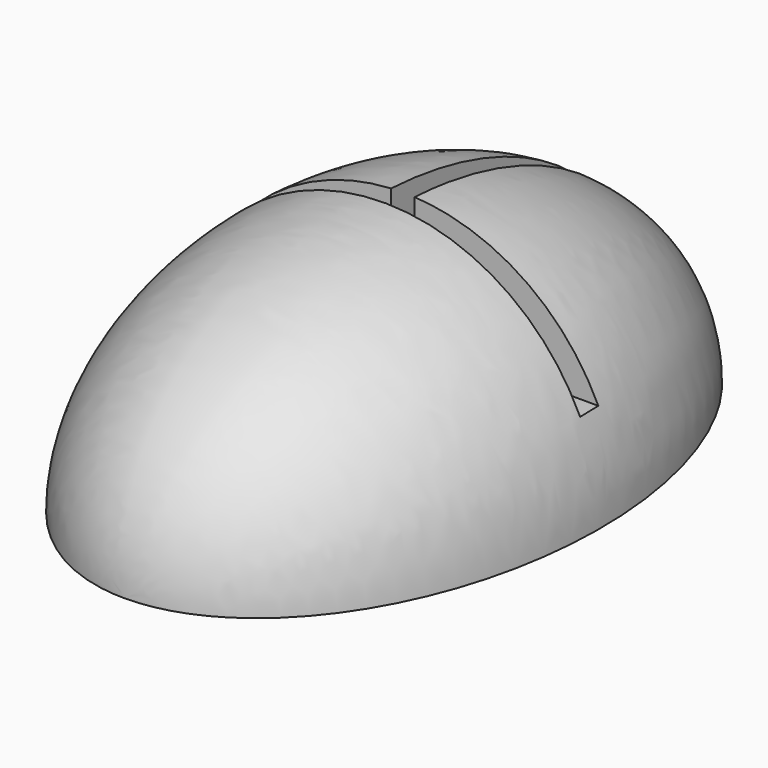
from build123d import *

# Parameters (mm, degrees)
F3_DEPTH      = 25
F3_DEPTH_BACK = 25
F5_START      = 1.48
F5_DEPTH      = 10.02


with BuildPart() as f1:
    # F0 (on Top) → F1 (revolve)
    with BuildSketch(Plane.XY):
        with BuildLine():
            Line((0, 1.8567474326), (0, 5.25))
            add(Edge.make_bspline(
                [(0, 5.25), (-3.5, 5.25), (-3.5, 0), (-3.5, -5.25), (0, -5.25)],
                knots=[0, 0, 0, 1.5707963268, 1.5707963268, 3.1415926536, 3.1415926536, 3.1415926536], degree=2, weights=[1, 0.7071067812, 1, 0.7071067812, 1]))
            Line((0, -5.25), (0, 0))
            Line((0, 0), (0, 1.8567474326))
        make_face()
    revolve(axis=Axis((0, 3.5533737163, 0), (0, 1, 0)))

    # F2 (on Right) → F3 (cut, two sides)
    with BuildSketch(Plane.YZ) as f3_sk:
        Polygon((6.3744364306, 0), (0, 0), (-6.297763437, 0), (-6.297763437, -3.5955796484), (6.3744364306, -3.5955796484), align=None)
    extrude(amount=-F3_DEPTH, mode=Mode.SUBTRACT)
    extrude(f3_sk.sketch, amount=F3_DEPTH_BACK, mode=Mode.SUBTRACT)

    # F4 (on Top) → F5 (cut)
    with BuildSketch(Plane.XY.offset(F5_START)):
        Polygon((-4.4482909143, 0), (0, 0), (4.5133754611, 0), (4.5133754611, 0.38), (0.1900000061, 0.38), (0.1900000061, 5.200644955), (0.1900000061, 5.4544974118), (-0.19, 5.4544974118), (-0.19, 5.200644955), (-0.19, 0.38), (-4.4482909143, 0.38), align=None)
    extrude(amount=F5_DEPTH, mode=Mode.SUBTRACT)


solid = f1.part
